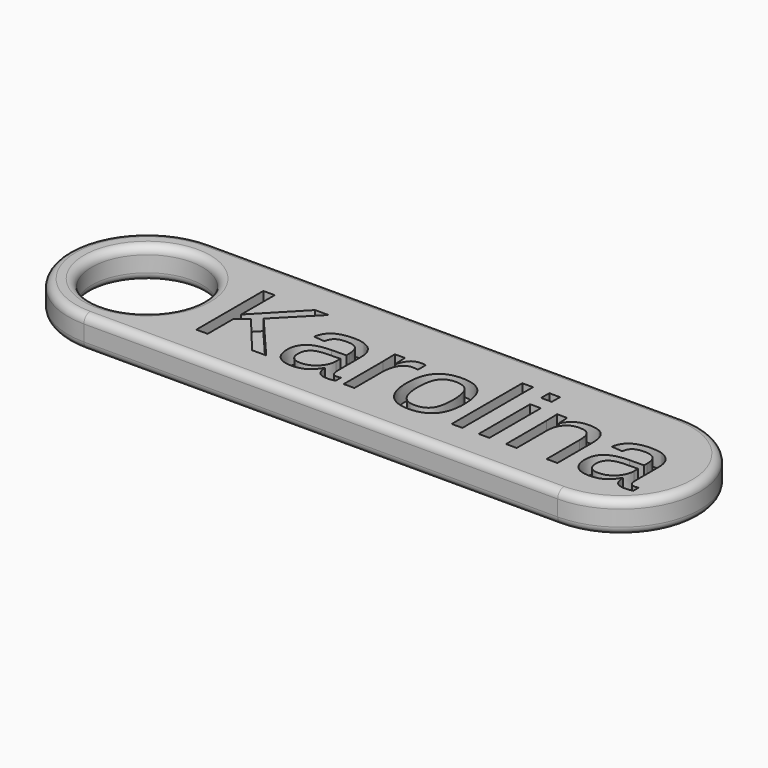
from build123d import *

# Parameters (mm, degrees)
F0_R         = 8.89
F1_DEPTH     = 5.08
F2_TEXT_SIZE = 19.5791666667
F3_DEPTH     = 2.54
F4_R         = 1.27


# Not quite as in the source:
# - Text() gives the source's letters only with a copy of the font that has no kerning and outlines rounded to 1/6400 em; it was checked with that copy


with BuildPart() as f1:
    # F0 (on Top) → F1 (new body)
    with BuildSketch(Plane.XY):
        with BuildLine():
            Line((-38.1, -12.7), (38.1, -12.7))
            ThreePointArc((38.1, -12.7), (50.8, 0), (38.1, 12.7))
            Line((38.1, 12.7), (-38.1, 12.7))
            ThreePointArc((-38.1, 12.7), (-50.8, 0), (-38.1, -12.7))
        make_face()
        with Locations((-38.1, 0)):
            Circle(F0_R, mode=Mode.SUBTRACT)
    extrude(amount=F1_DEPTH)

    # F2 (on face) → F3 (cut)
    with BuildSketch(Plane.XY.offset(5.08)):
        with Locations((-26.1993723958, -6.985)):
            Text('Karolina', F2_TEXT_SIZE, font='Arimo', text_align=(TextAlign.LEFT, TextAlign.BOTTOM))
    extrude(amount=-F3_DEPTH, mode=Mode.SUBTRACT)

    # F4
    f4_edges = [f1.edges().sort_by_distance(p)[0] for p in [
        (-50.8, 0, 5.08),
        (0, -12.7, 0),
        (50.8, 0, 0),
        (0, 12.7, 0),
        (-50.8, 0, 0),
        (-46.99, 0, 0),
        (-46.99, 0, 5.08),
    ]]
    fillet(f4_edges, radius=F4_R)


solid = f1.part
